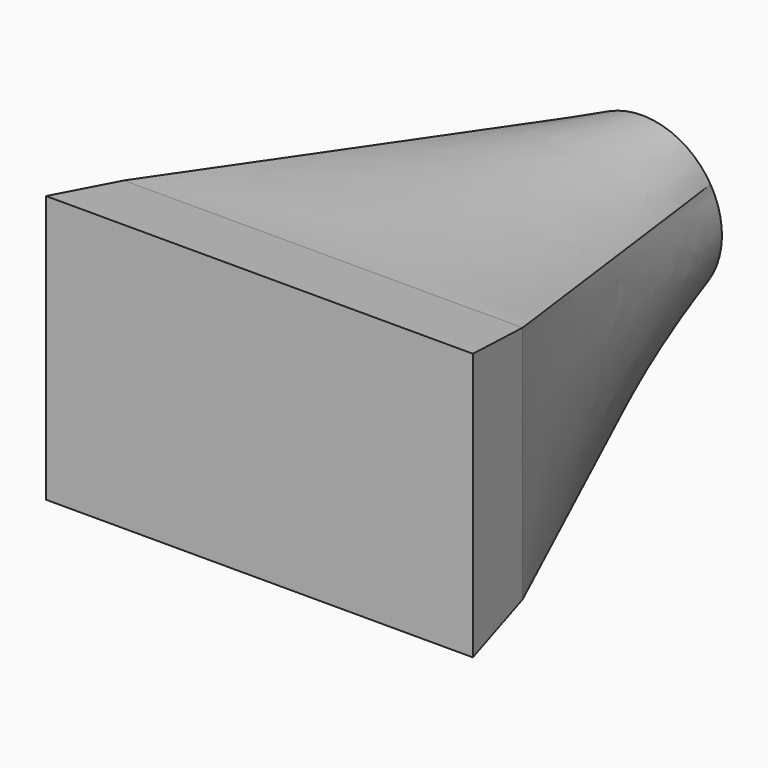
from build123d import *

# Parameters (mm, degrees)
F0_W      = 127
F0_H      = 76.2
F1_DEPTH  = 25.4
F1_TAPER  = -10
F1_FACE_W = 127
F1_FACE_H = 76.2


# Not quite as in the source:
# - the arcs of a loft's sections are written as splines that run evenly, so that the points pair up as in the source's solid


with BuildPart() as f1:
    # F0 (on Front) → F1 (new body)
    with BuildSketch(Plane.XZ):
        Rectangle(F0_W, F0_H)
    extrude(amount=F1_DEPTH, taper=F1_TAPER)

    # F1_face (on face) → F4 section 0
    with BuildSketch(Plane(origin=(0, 0, 0), x_dir=(1, 0, 0), z_dir=(0, 1, 0))):
        Rectangle(F1_FACE_W, F1_FACE_H)
    # F3 (on offset) → F4 section 1
    with BuildSketch(Plane(origin=(0, 127, 0), x_dir=(-1, 0, 0), z_dir=(0, 1, 0))):
        with BuildLine():
            add(Edge.make_bspline(
                [(-21.7803203131, 13.0681921879), (-22.6356314917, 11.6426735568), (-23.3505236623, 10.1329514593), (-24.472067113, 7.0029702123), (-24.8786906608, 5.3827884578), (-25.3680549193, 2.0941466499), (-25.4507835294, 0.4257679146), (-25.2891626016, -2.8951537939), (-25.04481706, -4.5476146508), (-24.2384219474, -7.773195101), (-23.6763923162, -9.3462349355), (-22.2562123309, -12.3525168797), (-21.3980970935, -13.7856846531), (-19.4187089559, -16.457138362), (-18.2974849998, -17.6953582406), (-15.8349554859, -19.9293212464), (-14.4937108189, -20.9250091345), (-13.0681921879, -21.7803203131)],
                knots=[0, 0, 0, 0, 0.125, 0.125, 0.25, 0.25, 0.375, 0.375, 0.5, 0.5, 0.625, 0.625, 0.75, 0.75, 0.875, 0.875, 1, 1, 1, 1], degree=3))
            add(Edge.make_bspline(
                [(-13.0681921879, -21.7803203131), (-11.6426735568, -22.6356314917), (-10.1329514593, -23.3505236623), (-7.0029702123, -24.472067113), (-5.3827884578, -24.8786906608), (-2.0941466499, -25.3680549193), (-0.4257679146, -25.4507835294), (2.8951537939, -25.2891626016), (4.5476146508, -25.04481706), (7.773195101, -24.2384219474), (9.3462349355, -23.6763923162), (12.3525168797, -22.2562123309), (13.7856846531, -21.3980970935), (16.457138362, -19.4187089559), (17.6953582406, -18.2974849998), (19.9293212464, -15.8349554859), (20.9250091345, -14.4937108189), (21.7803203131, -13.0681921879)],
                knots=[0, 0, 0, 0, 0.125, 0.125, 0.25, 0.25, 0.375, 0.375, 0.5, 0.5, 0.625, 0.625, 0.75, 0.75, 0.875, 0.875, 1, 1, 1, 1], degree=3))
            add(Edge.make_bspline(
                [(21.7803203131, -13.0681921879), (22.6356314917, -11.6426735568), (23.3505236623, -10.1329514593), (24.472067113, -7.0029702123), (24.8786906608, -5.3827884578), (25.3680549193, -2.0941466499), (25.4507835294, -0.4257679146), (25.2891626016, 2.8951537939), (25.04481706, 4.5476146508), (24.2384219474, 7.773195101), (23.6763923162, 9.3462349355), (22.2562123309, 12.3525168797), (21.3980970935, 13.7856846531), (19.4187089559, 16.457138362), (18.2974849998, 17.6953582406), (15.8349554859, 19.9293212464), (14.4937108189, 20.9250091345), (13.0681921879, 21.7803203131)],
                knots=[0, 0, 0, 0, 0.125, 0.125, 0.25, 0.25, 0.375, 0.375, 0.5, 0.5, 0.625, 0.625, 0.75, 0.75, 0.875, 0.875, 1, 1, 1, 1], degree=3))
            add(Edge.make_bspline(
                [(13.0681921879, 21.7803203131), (11.6426735568, 22.6356314917), (10.1329514593, 23.3505236623), (7.0029702123, 24.472067113), (5.3827884578, 24.8786906608), (2.0941466499, 25.3680549193), (0.4257679146, 25.4507835294), (-2.8951537939, 25.2891626016), (-4.5476146508, 25.04481706), (-7.773195101, 24.2384219474), (-9.3462349355, 23.6763923162), (-12.3525168797, 22.2562123309), (-13.7856846531, 21.3980970935), (-16.457138362, 19.4187089559), (-17.6953582406, 18.2974849998), (-19.9293212464, 15.8349554859), (-20.9250091345, 14.4937108189), (-21.7803203131, 13.0681921879)],
                knots=[0, 0, 0, 0, 0.125, 0.125, 0.25, 0.25, 0.375, 0.375, 0.5, 0.5, 0.625, 0.625, 0.75, 0.75, 0.875, 0.875, 1, 1, 1, 1], degree=3))
        make_face()
    loft(ruled=True)


solid = f1.part
